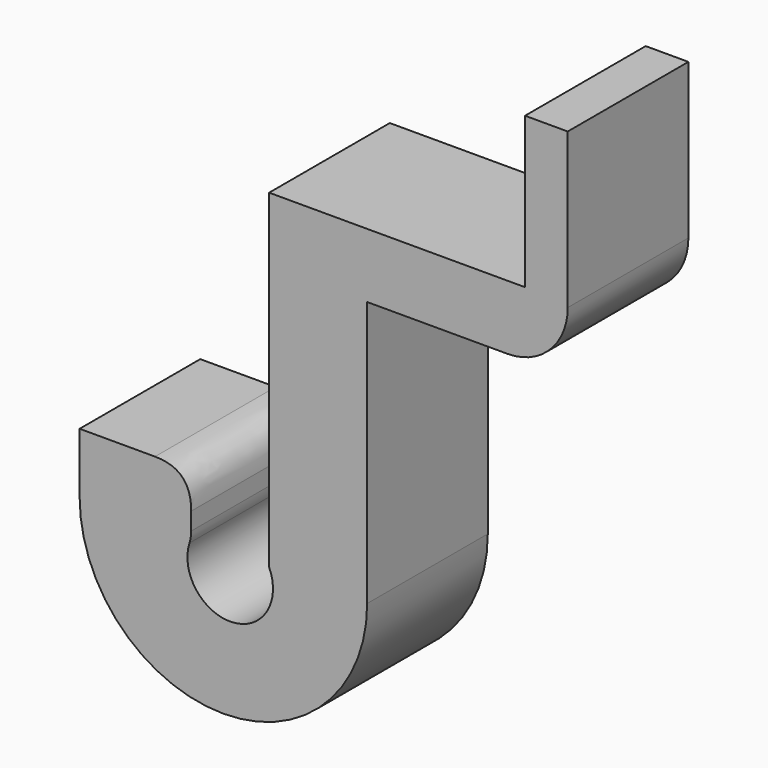
from build123d import *

# Parameters (mm, degrees)
F1_DEPTH    = 5
F2_R        = 2
F3_DEPTH    = 2
F4_T1_DEPTH = 11
F4_T3_DEPTH = 6.0917941426


# Not quite as in the source:
# - a fillet or chamfer that OpenCascade refuses, or shapes differently, is made with other operations: its cross-section is extruded or revolved along the edge and cut away or added


with BuildPart() as f1:
    # F0 (on Front) → F1 (new body)
    with BuildSketch(Plane.XZ):
        with BuildLine():
            Line((1.4157007724, 23.5682009265), (1.4157007724, 30.7082009265))
            Line((1.4157007724, 30.7082009265), (0, 30.7082009265))
            Line((0, 30.7082009265), (0, 29.0815811604))
            Line((0, 29.0815811604), (0, 25.7029440254))
            Line((0, 25.7029440254), (-8.4842955694, 25.7029440254))
            Line((-8.4842955694, 25.7029440254), (-8.4842955694, 14.7682009265))
            ThreePointArc((-8.4842955694, 14.7682009265), (-9.7762482479, 12.7647114857), (-11.0682009265, 14.7682009265))
            Line((-11.0682009265, 14.7682009265), (-14.7682009265, 14.7682009265))
            ThreePointArc((-14.7682009265, 14.7682009265), (-10.001250077, 10.001250077), (-5.2342992276, 14.7682009265))
            Line((-5.2342992276, 14.7682009265), (-5.2342992276, 23.5682009265))
            Line((-5.2342992276, 23.5682009265), (1.4157007724, 23.5682009265))
        make_face()
    extrude(amount=F1_DEPTH)

    # F2
    f2_edges = [f1.edges().sort_by_distance(p)[0] for p in [
        (1.415701, -2.5, 23.568201),
    ]]
    fillet(f2_edges, radius=F2_R)

    # F3 (add): a face of the model
    f3_faces = [f1.faces().sort_by_distance(p)[0] for p in [
        (-12.9182009265, -2.5, 14.7682009265),
    ]]
    extrude(f3_faces, amount=F3_DEPTH)

    # F4: fillet of radius 1.2 on 2 edges, made by hand

    # F4_s2 → F4_t1 (cut)
    with BuildSketch(Plane.XZ.offset(-3)):
        with BuildLine():
            add(Edge.make_bspline(
                [(-11.0682009265, 15.5682009265), (-11.0682009265, 16.7682009265), (-12.2682009265, 16.7682009265)],
                knots=[0, 0, 0, 1, 1, 1], degree=2, weights=[1, 1, 1]))
            Line((-12.2682009265, 16.7682009265), (-11.0682009265, 16.7682009265))
            Line((-11.0682009265, 16.7682009265), (-11.0682009265, 15.5682009265))
        make_face()
    extrude(amount=F4_T1_DEPTH, mode=Mode.SUBTRACT)

    # F4_s4 → F4_t3 (cut)
    with BuildSketch(Plane.XZ.offset(-0.5458970713)):
        with BuildLine():
            add(Edge.make_bspline(
                [(-11.1261089729, 14.6182854421), (-11.0682009265, 14.7978698213), (-11.0682009265, 14.986559755)],
                knots=[0, 0, 0, 1, 1, 1], degree=2, weights=[1, 1, 1]))
            Line((-11.0682009265, 14.986559755), (-11.0682009265, 14.7682009265))
            ThreePointArc((-11.0682009265, 14.7682009265), (-11.0992800608, 14.6940640537), (-11.1261089729, 14.6182854421))
        make_face()
    extrude(amount=F4_T3_DEPTH, mode=Mode.SUBTRACT)


solid = f1.part
